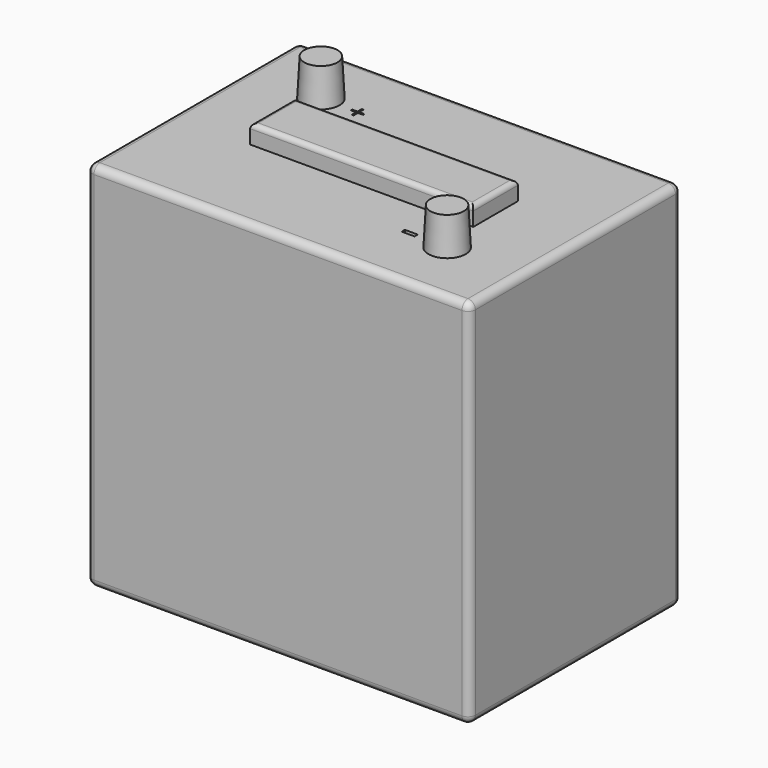
from build123d import *

# Parameters (mm, degrees)
F0_W           = 261.62
F0_H           = 254
F1_DEPTH       = 181.102
F2_R           = 5.08
F3_W           = 152.4
F3_H           = 38.1
F4_DEPTH       = 12.7
F3_R           = 12.7
F5_DEPTH       = 25.4
F5_TAPER       = 3
F6_R           = 3.175
F3_TEXT_SIZE   = 17.6388888889
F3_TEXT_SIZE_2 = 36.7450271248
F7_DEPTH       = 3.175


# Not quite as in the source:
# - Text() gives the source's letters only with a copy of the font that has no kerning and outlines rounded to 1/6400 em; it was checked with that copy


with BuildPart() as f1:
    # F0 (on Front) → F1 (new body)
    with BuildSketch(Plane.XZ):
        with Locations((-130.81, 127)):
            Rectangle(F0_W, F0_H)
    extrude(amount=F1_DEPTH)

    # F2
    f2_edges = [f1.edges().sort_by_distance(p)[0] for p in [
        (-130.81, -181.102, 0),
        (0, -181.102, 127),
        (-130.81, -181.102, 254),
        (-261.62, -181.102, 127),
        (0, -90.551, 254),
        (-261.62, -90.551, 254),
        (-130.81, 0, 254),
        (-130.81, 0, 0),
        (0, 0, 127),
        (-261.62, 0, 127),
        (-261.62, -90.551, 0),
        (0, -90.551, 0),
    ]]
    fillet(f2_edges, radius=F2_R)

    # F3 (on face) → F4 (join)
    with BuildSketch(Plane.XY.offset(254)):
        with Locations((-130.81, -90.551)):
            Rectangle(F3_W, F3_H)
    extrude(amount=F4_DEPTH)

    # F3 (on face) → F5 (join)
    with BuildSketch(Plane.XY.offset(254)):
        with Locations((-210.82, -44.45)):
            Circle(F3_R)
        with Locations((-50.8, -136.652)):
            Circle(F3_R)
    extrude(amount=F5_DEPTH, taper=F5_TAPER)

    # F6
    f6_edges = [f1.edges().sort_by_distance(p)[0] for p in [
        (-130.81, -71.501, 266.7),
        (-207.01, -90.551, 266.7),
        (-130.81, -109.601, 266.7),
        (-54.61, -90.551, 266.7),
    ]]
    fillet(f6_edges, radius=F6_R)

    # F3 (on face) → F7 (cut)
    with BuildSketch(Plane.XY.offset(254)):
        with Locations((-190.5779969618, -50.8)):
            Text('+', F3_TEXT_SIZE, font='Open Sans', text_align=(TextAlign.LEFT, TextAlign.BOTTOM))
        with Locations((-82.55, -146.177)):
            Text('-', F3_TEXT_SIZE_2, font='Open Sans', text_align=(TextAlign.LEFT, TextAlign.BOTTOM))
    extrude(amount=-F7_DEPTH, mode=Mode.SUBTRACT)


solid = f1.part
